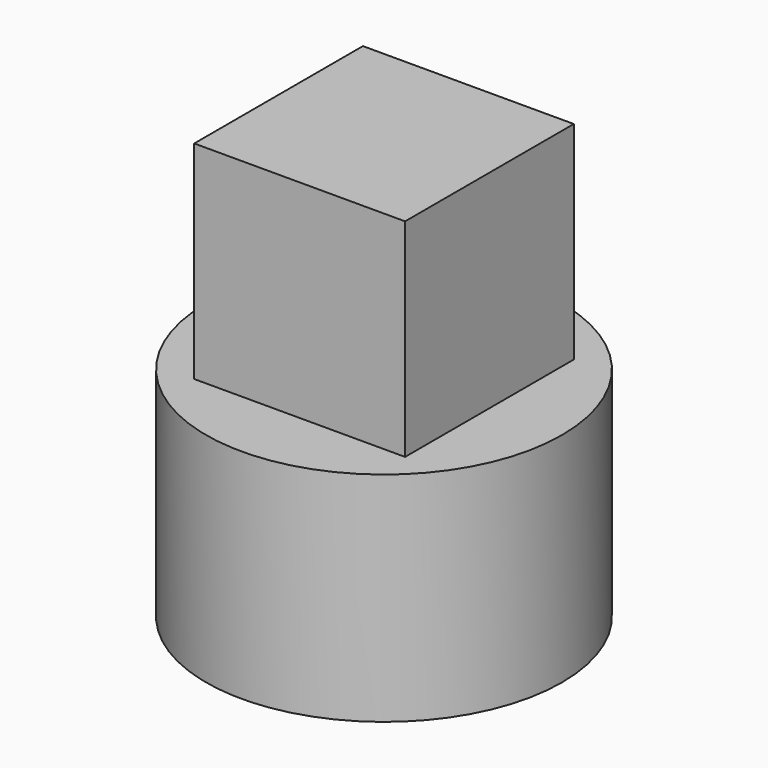
from build123d import *

# Parameters (mm, degrees)
F0_W     = 30.5
F0_H     = 30.5
F1_DEPTH = 30
F2_R     = 25.75
F2_W     = 30.5
F2_H     = 30.5
F2_R_2   = 15
F3_DEPTH = 1
F4_R     = 25.75
F4_R_2   = 15.4
F5_DEPTH = 30.5


# Not quite as in the source:
# - a feature names something its author has since deleted; it is built from what else it names


with BuildPart() as f1:
    # F0 (on Top) → F1 (new body)
    with BuildSketch(Plane.XY):
        Rectangle(F0_W, F0_H)
    extrude(amount=F1_DEPTH)

    # F2 (on face) → F3 (join)
    with BuildSketch(Plane(origin=(0, 0, 0), x_dir=(1, 0, 0), z_dir=(0, 0, -1))):
        Circle(F2_R)
        Rectangle(F2_W, F2_H, mode=Mode.SUBTRACT)
        Rectangle(F2_W, F2_H)
        Circle(F2_R_2, mode=Mode.SUBTRACT)
        Circle(F2_R_2)
    extrude(amount=F3_DEPTH)

    # F4 (on face) → F5 (join)
    with BuildSketch(Plane(origin=(0, 0, -1), x_dir=(1, 0, 0), z_dir=(0, 0, -1))):
        Circle(F4_R)
        Circle(F4_R_2, mode=Mode.SUBTRACT)
    extrude(amount=F5_DEPTH)


solid = f1.part
